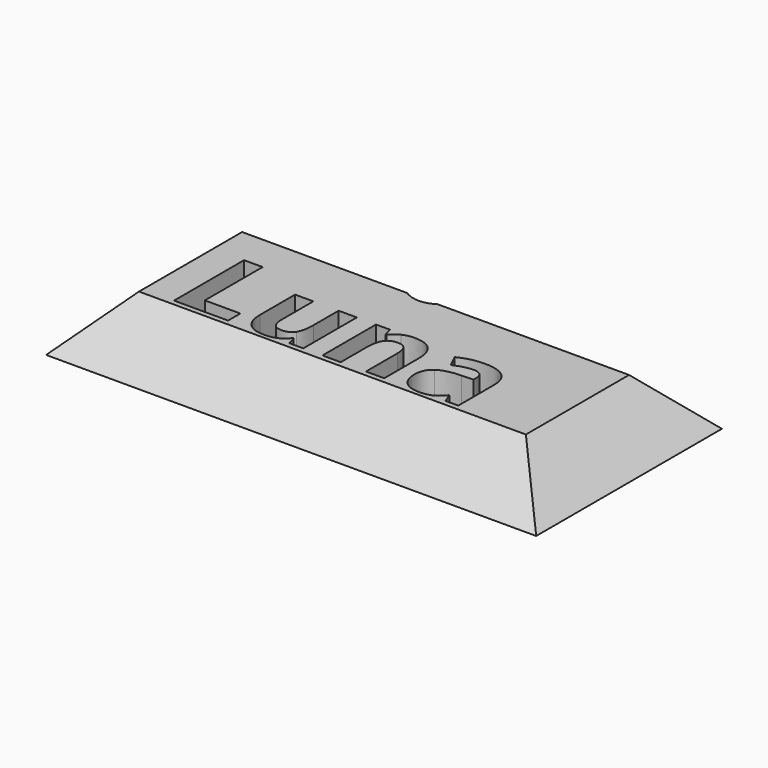
from build123d import *

# Parameters (mm, degrees)
F0_W        = 40
F0_H        = 20
F0_R        = 2.0889371437
F1_DEPTH    = 4
F2_T1_DEPTH = 65.7168298797
F2_T3_DEPTH = 45.7168298797


# Not quite as in the source:
# - a fillet or chamfer that OpenCascade refuses, or shapes differently, is made with other operations: its cross-section is extruded or revolved along the edge and cut away or added


with BuildPart() as f1:
    # F0 (on Top) → F1 (new body)
    with BuildSketch(Plane.XY):
        with Locations((20, 10)):
            Rectangle(F0_W, F0_H)
        Polygon((11.590113647, 5.4027722217), (7.3983091854, 5.4027722217), (7.3983091854, 12.1895739882), (8.8376637294, 12.1895739882), (8.8376637294, 6.5910938267), (11.590113647, 6.5910938267), align=None, mode=Mode.SUBTRACT)
        with BuildLine():
            Line((17.4203165215, 5.4027722217), (16.3344876549, 5.4027722217))
            Line((16.3344876549, 5.4027722217), (16.1443561981, 6.0667469185))
            Line((16.1443561981, 6.0667469185), (16.0700860978, 6.0667469185))
            add(Edge.make_bspline(
                [(16.0700860978, 6.0667469185), (15.8428195908, 5.704308829), (15.4246789261, 5.5067503622)],
                knots=[0, 0, 0, 1, 1, 1], degree=2))
            add(Edge.make_bspline(
                [(15.4246789261, 5.5067503622), (15.0065382613, 5.3091918953), (14.4732789411, 5.3091918953)],
                knots=[0, 0, 0, 1, 1, 1], degree=2))
            add(Edge.make_bspline(
                [(14.4732789411, 5.3091918953), (13.5582713053, 5.3091918953), (13.0940831783, 5.7993745574)],
                knots=[0, 0, 0, 1, 1, 1], degree=2))
            add(Edge.make_bspline(
                [(13.0940831783, 5.7993745574), (12.6298950514, 6.2895572194), (12.6298950514, 7.2090210613)],
                knots=[0, 0, 0, 1, 1, 1], degree=2))
            Line((12.6298950514, 7.2090210613), (12.6298950514, 10.5927668315))
            Line((12.6298950514, 10.5927668315), (14.0454831633, 10.5927668315))
            Line((14.0454831633, 10.5927668315), (14.0454831633, 7.5610613368))
            add(Edge.make_bspline(
                [(14.0454831633, 7.5610613368), (14.0454831633, 6.9995793784), (14.2452697331, 6.7188383992)],
                knots=[0, 0, 0, 1, 1, 1], degree=2))
            add(Edge.make_bspline(
                [(14.2452697331, 6.7188383992), (14.445056303, 6.4380974201), (14.8817644928, 6.4380974201)],
                knots=[0, 0, 0, 1, 1, 1], degree=2))
            add(Edge.make_bspline(
                [(14.8817644928, 6.4380974201), (15.4759252953, 6.4380974201), (15.7403268524, 6.8346997557)],
                knots=[0, 0, 0, 1, 1, 1], degree=2))
            add(Edge.make_bspline(
                [(15.7403268524, 6.8346997557), (16.0047284095, 7.2313020914), (16.0047284095, 8.1507659333)],
                knots=[0, 0, 0, 1, 1, 1], degree=2))
            Line((16.0047284095, 8.1507659333), (16.0047284095, 10.5927668315))
            Line((16.0047284095, 10.5927668315), (17.4203165215, 10.5927668315))
            Line((17.4203165215, 10.5927668315), (17.4203165215, 5.4027722217))
        make_face(mode=Mode.SUBTRACT)
        with BuildLine():
            Line((23.6961399978, 8.7865179919), (23.6961399978, 5.4027722217))
            Line((23.6961399978, 5.4027722217), (22.2805518859, 5.4027722217))
            Line((22.2805518859, 5.4027722217), (22.2805518859, 8.4344777164))
            add(Edge.make_bspline(
                [(22.2805518859, 8.4344777164), (22.2805518859, 8.9959596748), (22.080765316, 9.276700654)],
                knots=[0, 0, 0, 1, 1, 1], degree=2))
            add(Edge.make_bspline(
                [(22.080765316, 9.276700654), (21.8809787462, 9.5574416332), (21.4442705564, 9.5574416332)],
                knots=[0, 0, 0, 1, 1, 1], degree=2))
            add(Edge.make_bspline(
                [(21.4442705564, 9.5574416332), (20.8501097539, 9.5574416332), (20.5857081968, 9.1608392975)],
                knots=[0, 0, 0, 1, 1, 1], degree=2))
            add(Edge.make_bspline(
                [(20.5857081968, 9.1608392975), (20.3213066396, 8.7642369618), (20.3213066396, 7.84477312)],
                knots=[0, 0, 0, 1, 1, 1], degree=2))
            Line((20.3213066396, 7.84477312), (20.3213066396, 5.4027722217))
            Line((20.3213066396, 5.4027722217), (18.9057185277, 5.4027722217))
            Line((18.9057185277, 5.4027722217), (18.9057185277, 10.5927668315))
            Line((18.9057185277, 10.5927668315), (19.9870911882, 10.5927668315))
            Line((19.9870911882, 10.5927668315), (20.177222645, 9.9287921347))
            Line((20.177222645, 9.9287921347), (20.2559489514, 9.9287921347))
            add(Edge.make_bspline(
                [(20.2559489514, 9.9287921347), (20.4936132724, 10.3045988423), (20.9087831331, 10.4969584021)],
                knots=[0, 0, 0, 1, 1, 1], degree=2))
            add(Edge.make_bspline(
                [(20.9087831331, 10.4969584021), (21.3239529939, 10.6893179619), (21.8527561081, 10.6893179619)],
                knots=[0, 0, 0, 1, 1, 1], degree=2))
            add(Edge.make_bspline(
                [(21.8527561081, 10.6893179619), (22.7588513319, 10.6893179619), (23.2274956648, 10.1998780009)],
                knots=[0, 0, 0, 1, 1, 1], degree=2))
            add(Edge.make_bspline(
                [(23.2274956648, 10.1998780009), (23.6961399978, 9.7104380398), (23.6961399978, 8.7865179919)],
                knots=[0, 0, 0, 1, 1, 1], degree=2))
        make_face(mode=Mode.SUBTRACT)
        with BuildLine():
            Line((29.4372187519, 5.4027722217), (28.4494264178, 5.4027722217))
            Line((28.4494264178, 5.4027722217), (28.1746270466, 6.1083381747))
            Line((28.1746270466, 6.1083381747), (28.1374919965, 6.1083381747))
            add(Edge.make_bspline(
                [(28.1374919965, 6.1083381747), (27.780995515, 5.6582613668), (27.4022180034, 5.4837266311)],
                knots=[0, 0, 0, 1, 1, 1], degree=2))
            add(Edge.make_bspline(
                [(27.4022180034, 5.4837266311), (27.0234404918, 5.3091918953), (26.4159110712, 5.3091918953)],
                knots=[0, 0, 0, 1, 1, 1], degree=2))
            add(Edge.make_bspline(
                [(26.4159110712, 5.3091918953), (25.6687538621, 5.3091918953), (25.2394726823, 5.7369876731)],
                knots=[0, 0, 0, 1, 1, 1], degree=2))
            add(Edge.make_bspline(
                [(25.2394726823, 5.7369876731), (24.8101915025, 6.1647834509), (24.8101915025, 6.9535319162)],
                knots=[0, 0, 0, 1, 1, 1], degree=2))
            add(Edge.make_bspline(
                [(24.8101915025, 6.9535319162), (24.8101915025, 7.7794154317), (25.3880128829, 8.1715615613)],
                knots=[0, 0, 0, 1, 1, 1], degree=2))
            add(Edge.make_bspline(
                [(25.3880128829, 8.1715615613), (25.9658342633, 8.563707691), (27.1303894362, 8.6052989472)],
                knots=[0, 0, 0, 1, 1, 1], degree=2))
            Line((27.1303894362, 8.6052989472), (28.032028454, 8.6335215853))
            Line((28.032028454, 8.6335215853), (28.032028454, 8.8607880922))
            add(Edge.make_bspline(
                [(28.032028454, 8.8607880922), (28.032028454, 9.6495365575), (27.2239697626, 9.6495365575)],
                knots=[0, 0, 0, 1, 1, 1], degree=2))
            add(Edge.make_bspline(
                [(27.2239697626, 9.6495365575), (26.601586322, 9.6495365575), (25.7608487865, 9.27372985)],
                knots=[0, 0, 0, 1, 1, 1], degree=2))
            Line((25.7608487865, 9.27372985), (25.2929471545, 10.230328742))
            add(Edge.make_bspline(
                [(25.2929471545, 10.230328742), (26.1886445643, 10.699715776), (27.2789296369, 10.699715776)],
                knots=[0, 0, 0, 1, 1, 1], degree=2))
            add(Edge.make_bspline(
                [(27.2789296369, 10.699715776), (28.3231672472, 10.699715776), (28.8801929996, 10.244440061)],
                knots=[0, 0, 0, 1, 1, 1], degree=2))
            add(Edge.make_bspline(
                [(28.8801929996, 10.244440061), (29.4372187519, 9.7891643461), (29.4372187519, 8.8607880922)],
                knots=[0, 0, 0, 1, 1, 1], degree=2))
            Line((29.4372187519, 8.8607880922), (29.4372187519, 5.4027722217))
        make_face(mode=Mode.SUBTRACT)
        with Locations((18.9712941647, 16.7298167944)):
            Circle(F0_R, mode=Mode.SUBTRACT)
    extrude(amount=F1_DEPTH)

    # F2: chamfer of 5 on 4 edges, made by hand

    # F2_s2 → F2_t1 (cut)
    with BuildSketch(Plane.YZ.offset(-12.8584149398)):
        Polygon((20, -1), (15, 4), (20, 4), align=None)
        Polygon((0, -1), (5, 4), (0, 4), align=None)
    extrude(amount=F2_T1_DEPTH, mode=Mode.SUBTRACT)

    # F2_s4 → F2_t3 (cut)
    with BuildSketch(Plane.XZ.offset(-32.8584149398)):
        Polygon((0, -1), (5, 4), (0, 4), align=None)
        Polygon((40, -1), (35, 4), (40, 4), align=None)
    extrude(amount=F2_T3_DEPTH, mode=Mode.SUBTRACT)


solid = f1.part
